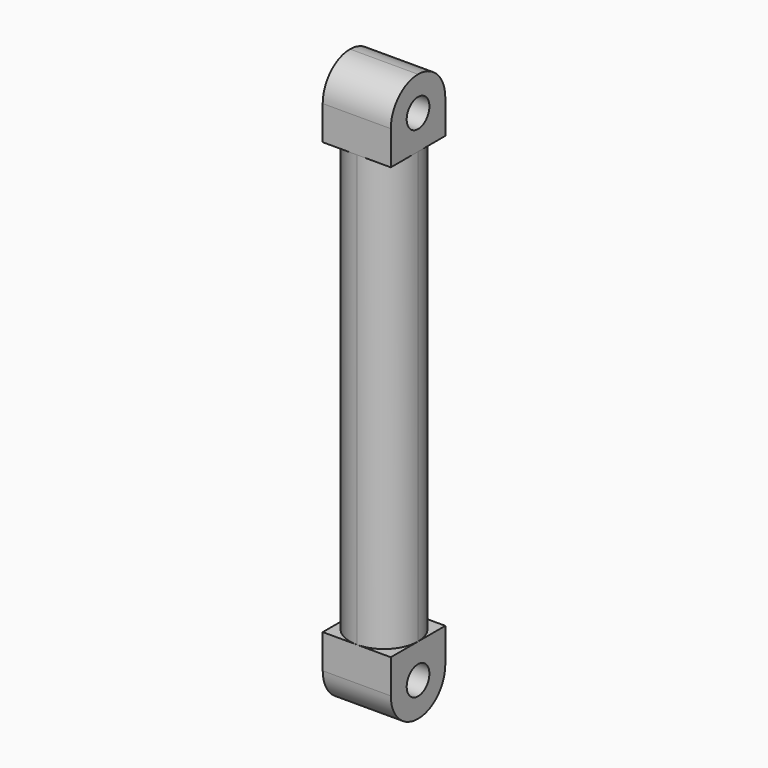
from build123d import *

# Parameters (mm, degrees)
F0_R     = 1.25
F1_DEPTH = 6
F2_DEPTH = 44
F3_R     = 1.25
F4_DEPTH = 6
F5_W     = 6
F5_H     = 6
F6_DEPTH = 6
F7_R     = 1.25
F8_DEPTH = 25


# Not quite as in the source:
# - a feature names something its author has since deleted; it is built from what else it names


with BuildPart() as f1:
    # F0 (on Top) → F1 (new body)
    with BuildSketch(Plane.XY):
        with BuildLine():
            ThreePointArc((0, -3), (2.1213203436, -2.1213203436), (3, 0))
            ThreePointArc((3, 0), (2.1213203436, 2.1213203436), (0, 3))
            ThreePointArc((0, 3), (-2.1213203436, 2.1213203436), (-3, 0))
            ThreePointArc((-3, 0), (-2.1213203436, -2.1213203436), (0, -3))
        make_face()
        Circle(F0_R, mode=Mode.SUBTRACT)
        with BuildLine():
            ThreePointArc((-3, 0), (-2.1213203436, 2.1213203436), (0, 3))
            Line((0, 3), (-3, 3))
            Line((-3, 3), (-3, 0))
        make_face()
        with BuildLine():
            Line((-3, -3), (0, -3))
            ThreePointArc((0, -3), (-2.1213203436, -2.1213203436), (-3, 0))
            Line((-3, 0), (-3, -3))
        make_face()
        with BuildLine():
            Line((3, -3), (3, 0))
            ThreePointArc((3, 0), (2.1213203436, -2.1213203436), (0, -3))
            Line((0, -3), (3, -3))
        make_face()
        with BuildLine():
            ThreePointArc((0, 3), (2.1213203436, 2.1213203436), (3, 0))
            Line((3, 0), (3, 3))
            Line((3, 3), (0, 3))
        make_face()
        Circle(F0_R)
    extrude(amount=F1_DEPTH)

    # F0 (on Top) → F2 (join)
    with BuildSketch(Plane.XY):
        with BuildLine():
            ThreePointArc((0, -3), (2.1213203436, -2.1213203436), (3, 0))
            ThreePointArc((3, 0), (2.1213203436, 2.1213203436), (0, 3))
            ThreePointArc((0, 3), (-2.1213203436, 2.1213203436), (-3, 0))
            ThreePointArc((-3, 0), (-2.1213203436, -2.1213203436), (0, -3))
        make_face()
        Circle(F0_R, mode=Mode.SUBTRACT)
    extrude(amount=F2_DEPTH)

    # F3 (on face) → F4 (cut)
    with BuildSketch(Plane.YZ.offset(3)):
        with Locations((0, 3)):
            Circle(F3_R)
        with BuildLine():
            Line((-3, 0), (0, 0))
            ThreePointArc((0, 0), (-2.1213203436, 0.8786796564), (-3, 3))
            Line((-3, 3), (-3, 0))
        make_face()
        with BuildLine():
            Line((3, 0), (3, 3))
            ThreePointArc((3, 3), (2.1213203436, 0.8786796564), (0, 0))
            Line((0, 0), (3, 0))
        make_face()
    extrude(amount=-F4_DEPTH, mode=Mode.SUBTRACT)

    # F5 (on face) → F6 (join)
    with BuildSketch(Plane.XY.offset(44)):
        Rectangle(F5_W, F5_H)
    extrude(amount=F6_DEPTH)

    # F7 (on face) → F8 (cut)
    with BuildSketch(Plane.YZ.offset(3)):
        with Locations((0, 47)):
            Circle(F7_R)
        with BuildLine():
            Line((-3, 50), (-3, 47))
            ThreePointArc((-3, 47), (-2.1213203436, 49.1213203436), (0, 50))
            Line((0, 50), (-3, 50))
        make_face()
        with BuildLine():
            ThreePointArc((0, 50), (2.1213203436, 49.1213203436), (3, 47))
            Line((3, 47), (3, 50))
            Line((3, 50), (0, 50))
        make_face()
    extrude(amount=-F8_DEPTH, mode=Mode.SUBTRACT)


solid = f1.part
